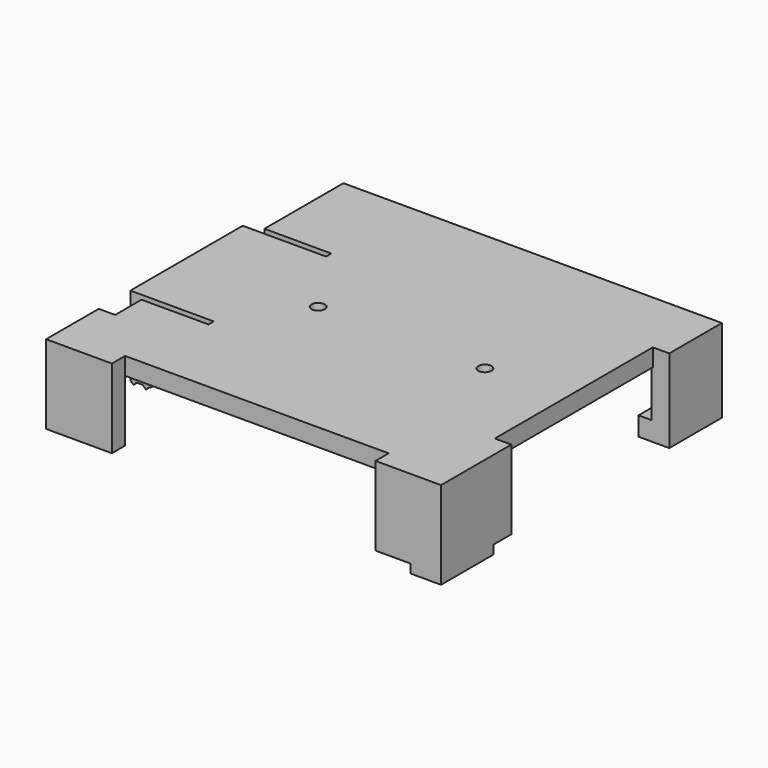
from build123d import *

# Parameters (mm, degrees)
F0_W      = 90
F0_H      = 80
F1_DEPTH  = 4
F2_R      = 1.5
F3_DEPTH  = 4.001
F5_DEPTH  = 14
F6_W      = 7
F6_H      = 15
F7_DEPTH  = 2
F8_W      = 3.75
F8_H      = 60
F9_DEPTH  = 2
F10_W     = 3.75
F10_H     = 15
F10_W_2   = 3.25
F11_DEPTH = 3
F12_W     = 3.75
F12_H     = 45
F13_DEPTH = 16.001
F14_W     = 19
F14_H     = 1.5
F15_DEPTH = 25
F16_W     = 3.75
F16_H     = 22.5
F17_DEPTH = 25
F18_W     = 32
F18_H     = 2
F19_DEPTH = 1.5
F20_R     = 1
F21_W     = 1.4166666667
F21_H     = 32
F22_DEPTH = 0.7085
F23_SIZE  = 0.7075
F24_SIZE  = 1.8
F25_W     = 3.75
F25_H     = 7.5
F25_W_2   = 60.0602255464
F25_H_2   = 3.75
F26_DEPTH = 25
F27_W     = 15.25
F27_H     = 32
F28_DEPTH = 1.5
F29_W     = 32
F29_H     = 13.5
F30_DEPTH = 0.3
F31_W     = 3.25
F31_H     = 15
F32_DEPTH = 1.3
F33_W     = 15
F33_H     = 10.7
F34_DEPTH = 0.3
F35_W     = 1.2
F35_H     = 32
F36_DEPTH = 1
F37_R     = 1.19999


# Not quite as in the source:
# - a fillet or chamfer is up to 0.001 mm smaller than in the source, because OpenCascade refuses the exact size
# - a feature names something its author has since deleted; it is built from what else it names


with BuildPart() as f1:
    # F0 (on Top) → F1 (new body)
    with BuildSketch(Plane.XY):
        Rectangle(F0_W, F0_H)
    extrude(amount=F1_DEPTH)

    # F2 (on face) → F3 (cut, through all)
    with BuildSketch(Plane.XY.offset(4)):
        with Locations((23, 0)):
            Circle(F2_R)
        with Locations((-15, 0)):
            Circle(F2_R)
    extrude(amount=-F3_DEPTH, mode=Mode.SUBTRACT)

    # F4 (on face) → F5 (join)
    with BuildSketch(Plane(origin=(0, 0, 0), x_dir=(1, 0, 0), z_dir=(0, 0, -1))):
        Polygon((-41.25, -36.25), (-41.25, 36.25), (-30, 36.25), (-30, 40), (-45, 40), (-45, -40), (-41.25, -40), align=None)
        Polygon((45, 40), (30, 40), (30, 36.25), (41.25, 36.25), (41.25, -36.25), (41.25, -40), (45, -40), align=None)
    extrude(amount=F5_DEPTH)

    # F6 (on face) → F7 (join)
    with BuildSketch(Plane(origin=(0, 0, -14), x_dir=(1, 0, 0), z_dir=(0, 0, -1))):
        with Locations((41.5, 32.5)):
            Rectangle(F6_W, F6_H)
    extrude(amount=F7_DEPTH)

    # F8 (on face) → F9 (cut)
    with BuildSketch(Plane(origin=(0, 0, -14), x_dir=(1, 0, 0), z_dir=(0, 0, -1))):
        with Locations((43.125, -10)):
            Rectangle(F8_W, F8_H)
    extrude(amount=-F9_DEPTH, mode=Mode.SUBTRACT)

    # F10 (on face) → F11 (join)
    with BuildSketch(Plane(origin=(0, 0, -12), x_dir=(1, 0, 0), z_dir=(0, 0, -1))):
        with Locations((43.125, -32.5)):
            Rectangle(F10_W, F10_H)
        with Locations((39.625, -32.5)):
            Rectangle(F10_W_2, F10_H)
    extrude(amount=F11_DEPTH)

    # F12 (on face) → F13 (cut, through all)
    with BuildSketch(Plane(origin=(0, 0, -12), x_dir=(1, 0, 0), z_dir=(0, 0, -1))):
        with Locations((43.125, -2.5)):
            Rectangle(F12_W, F12_H)
    extrude(amount=-F13_DEPTH, mode=Mode.SUBTRACT)

    # F14 (on face) → F15 (cut)
    with BuildSketch(Plane(origin=(0, 0, -14), x_dir=(1, 0, 0), z_dir=(0, 0, -1))):
        with Locations((-35.5, 16.75)):
            Rectangle(F14_W, F14_H)
        with Locations((-35.5, -16.75)):
            Rectangle(F14_W, F14_H)
    extrude(amount=-F15_DEPTH, mode=Mode.SUBTRACT)

    # F16 (on face) → F17 (cut)
    with BuildSketch(Plane(origin=(0, 0, -14), x_dir=(1, 0, 0), z_dir=(0, 0, -1))):
        with Locations((-43.125, -28.75)):
            Rectangle(F16_W, F16_H)
    extrude(amount=-F17_DEPTH, mode=Mode.SUBTRACT)

    # F18 (on face) → F19 (join)
    with BuildSketch(Plane.YZ.offset(-41.25)):
        with Locations((0, -13)):
            Rectangle(F18_W, F18_H)
    extrude(amount=F19_DEPTH)

    # F20
    f20_edges = [f1.edges().sort_by_distance(p)[0] for p in [
        (-39.75, 0, -14),
    ]]
    fillet(f20_edges, radius=F20_R)

    # F21 (on face) → F22 (join)
    with BuildSketch(Plane(origin=(0, 0, -14), x_dir=(1, 0, 0), z_dir=(0, 0, -1))):
        with Locations((-41.4583333333, 0)):
            Rectangle(F21_W, F21_H)
        with Locations((-44.2916666667, 0)):
            Rectangle(F21_W, F21_H)
    extrude(amount=F22_DEPTH)

    # F23 (size 0.7085 in the source; OpenCascade refuses exactly that, so slightly less here)
    f23_edges = [f1.edges().sort_by_distance(p)[0] for p in [
        (-40.75, 0, -14.7085),
        (-42.166667, 0, -14.7085),
        (-43.583333, 0, -14.7085),
        (-45, 0, -14.7085),
    ]]
    chamfer(f23_edges, length=F23_SIZE)

    # F24
    f24_edges = [f1.edges().sort_by_distance(p)[0] for p in [
        (-16.5, 0, 0),
        (21.5, 0, 0),
    ]]
    chamfer(f24_edges, length=F24_SIZE)

    # F25 (on face) → F26 (cut)
    with BuildSketch(Plane(origin=(0, 0, -14), x_dir=(1, 0, 0), z_dir=(0, 0, -1))):
        with Locations((-43.125, 21.25)):
            Rectangle(F25_W, F25_H)
        with Locations((0.0301127732, 38.125)):
            Rectangle(F25_W_2, F25_H_2)
    extrude(amount=-F26_DEPTH, mode=Mode.SUBTRACT)

    # F27 (on face) → F28 (cut)
    with BuildSketch(Plane(origin=(0, 0, 0), x_dir=(1, 0, 0), z_dir=(0, 0, -1))):
        with Locations((-33.625, 0)):
            Rectangle(F27_W, F27_H)
    extrude(amount=-F28_DEPTH, mode=Mode.SUBTRACT)

    # F29 (on face) → F30 (join)
    with BuildSketch(Plane.YZ.offset(-41.25)):
        with Locations((0, -5.25)):
            Rectangle(F29_W, F29_H)
    extrude(amount=F30_DEPTH)

    # F31 (on face) → F32 (join)
    with BuildSketch(Plane.XY.offset(-12)):
        with Locations((39.625, 32.5)):
            Rectangle(F31_W, F31_H)
    extrude(amount=F32_DEPTH)

    # F33 (on face) → F34 (join)
    with BuildSketch(Plane(origin=(41.25, 0, 0), x_dir=(0, -1, 0), z_dir=(-1, 0, 0))):
        with Locations((-32.5, -5.35)):
            Rectangle(F33_W, F33_H)
    extrude(amount=F34_DEPTH)

    # F35 (on face) → F36 (join)
    with BuildSketch(Plane.XY.offset(-12)):
        with Locations((-40.35, 0)):
            Rectangle(F35_W, F35_H)
    extrude(amount=F36_DEPTH)

    # F37 (radius 1.2 in the source; OpenCascade refuses exactly that, so slightly less here)
    f37_edges = [f1.edges().sort_by_distance(p)[0] for p in [
        (-39.75, 0, -11),
    ]]
    fillet(f37_edges, radius=F37_R)


solid = f1.part
